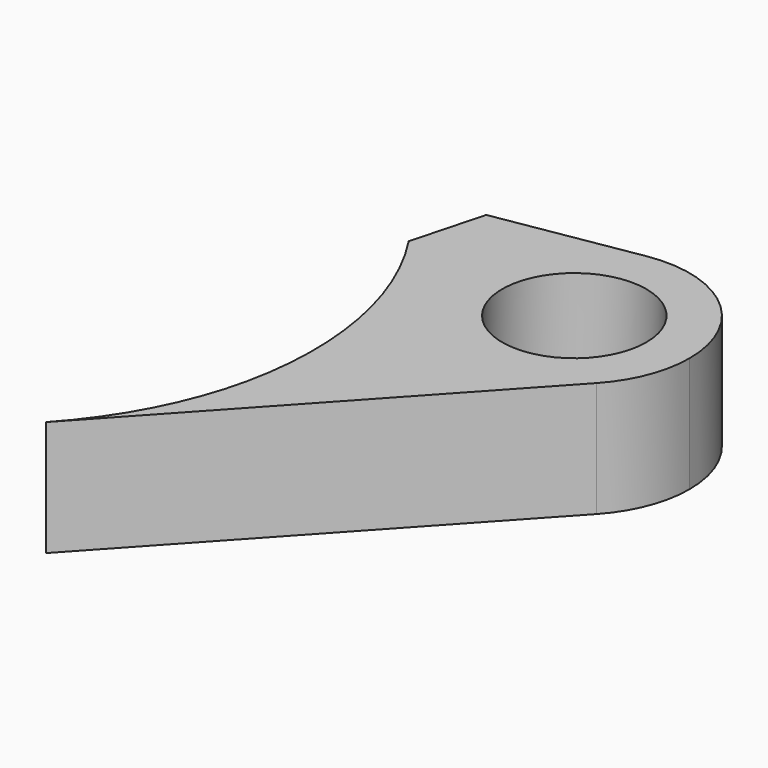
from build123d import *

# Parameters (mm, degrees)
F0_R     = 7.9375
F1_DEPTH = 12.7


with BuildPart() as f1:
    # F0 (on Top) → F1 (new body)
    with BuildSketch(Plane.XY):
        with BuildLine():
            ThreePointArc((31.8073335192, 20.9738774288), (37.4513031941, 7.0007063262), (37.2360288719, -8.0677229656))
            ThreePointArc((37.2360288719, -8.0677229656), (33.9725367984, -17.0138251575), (28.4983711579, -24.8059131627))
            Line((28.4983711579, -24.8059131627), (60.9339033423, 10.4515771637))
            ThreePointArc((60.9339033423, 10.4515771637), (40.4207699943, 13.0005062761), (49.4900105586, 31.5756120621))
            Line((49.4900105586, 31.5756120621), (33.9508555908, 28.9736107071))
            Line((33.9508555908, 28.9736107071), (31.8073335192, 20.9738774288))
        make_face()
        with BuildLine():
            ThreePointArc((49.4900105586, 31.5756120621), (40.4207699943, 13.0005062761), (60.9339033423, 10.4515771637))
            ThreePointArc((60.9339033423, 10.4515771637), (63.4193607937, 14.4353815135), (64.2874, 19.05))
            ThreePointArc((64.2874, 19.05), (59.79267739, 28.7434732141), (49.4900105586, 31.5756120621))
        make_face()
        with Locations((51.5874, 19.05)):
            Circle(F0_R, mode=Mode.SUBTRACT)
    extrude(amount=F1_DEPTH)


solid = f1.part
